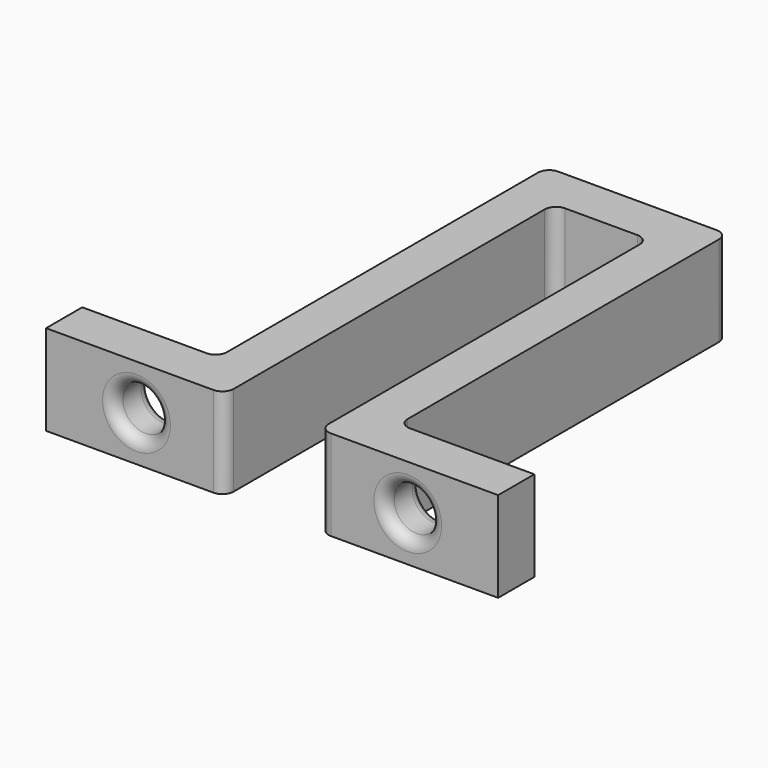
from build123d import *

# Parameters (mm, degrees)
F2_DEPTH = 4
F1_R     = 1
F3_DEPTH = 22.2
F5_R     = 0.49999


# Not quite as in the source:
# - a fillet or chamfer is up to 0.001 mm smaller than in the source, because OpenCascade refuses the exact size


with BuildPart() as f2:
    # F0 (on Top) → F2 (new body)
    with BuildSketch(Plane.XY):
        Polygon((0, 2), (0, 0), (7.9, 0), (7.9, 18.2000004202), (12.1, 18.2000004202), (12.1, 0), (20, 0), (20, 2), (14, 2), (14, 20.2), (6, 20.2), (6, 2), align=None)
    extrude(amount=F2_DEPTH)


with BuildPart() as f3:
    # F1 (on Front) → F3 (new body)
    with BuildSketch(Plane.XZ):
        with Locations((4, 2)):
            Circle(F1_R)
    extrude(amount=-F3_DEPTH)


with BuildPart() as f3b:
    # F1 (on Front) → F3, piece 2 (new body)
    with BuildSketch(Plane.XZ):
        with Locations((16, 2)):
            Circle(F1_R)
    extrude(amount=-F3_DEPTH)


with BuildPart() as f2_1:
    add(f2.part)

    # F4: cut F3, F3b
    add(f3.part, mode=Mode.SUBTRACT)
    add(f3b.part, mode=Mode.SUBTRACT)

    # F5 (radius 0.5 in the source; OpenCascade refuses exactly that, so slightly less here)
    f5_edges = [f2_1.edges().sort_by_distance(p)[0] for p in [
        (7.9, 0, 2),
        (12.1, 0, 2),
        (14, 20.2, 2),
        (7.9, 18.2, 2),
        (12.1, 18.2, 2),
        (6, 20.2, 2),
        (6, 2, 2),
        (14, 2, 2),
        (3, 2, 2),
        (15, 2, 2),
        (3, 0, 2),
        (15, 0, 2),
    ]]
    fillet(f5_edges, radius=F5_R)


solid = f2_1.part
